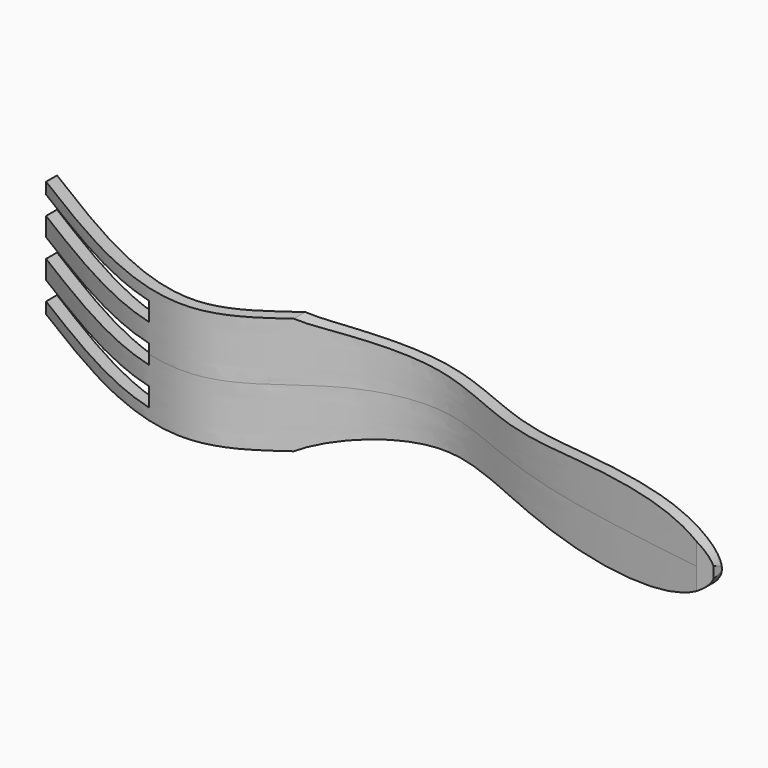
from build123d import *

# Parameters (mm, degrees)
F1_DEPTH = 12.7
F3_DEPTH = 25.4


# Not quite as in the source:
# - the dataset's text gives a spline's control points without its knots; the knots are read off the source's solid


with BuildPart() as f1:
    # F0 (on Top) → F1 (new body, symmetric)
    with BuildSketch(Plane.XY):
        with BuildLine():
            add(Edge.make_bspline(
                [(0, 0), (16.2681023426, -9.9387943725), (47.2246723498, -29.7831151482), (66.4369579208, -8.871840766), (90.9937113299, -1.8855664984), (116.1887648178, -16.7799469051), (146.2514664221, -20.7702417622), (163.4278756793, -23.4379916155)],
                knots=[0, 0, 0, 0, 0.2483058837, 0.4138785293, 0.5787286939, 0.7596256652, 1, 1, 1, 1], degree=3))
            Line((0, 0), (-1.3242090893, -2.1675032383))
            add(Edge.make_bspline(
                [(-1.3242090893, -2.1675032383), (2.7614631736, -4.6635937864), (9.136853643, -8.6121295805), (17.7262559137, -13.5899705503), (24.1194299019, -17.0078501308), (30.3765559587, -19.9378210176), (35.4147953662, -21.8277076646), (39.3127764924, -22.9151398196), (42.1656931351, -23.4919098932), (44.48213371, -23.7484534526), (46.2950869864, -23.8013359281), (47.6370394902, -23.7589266462), (48.9432550214, -23.6315977539), (50.6317203365, -23.3574905101), (52.6439135321, -22.8337162857), (54.9048810043, -21.9693426121), (57.7345292676, -20.5748674665), (60.9787182767, -18.5076431259), (63.9993416883, -16.3025670539), (66.3702951088, -14.6082956793), (68.14443987, -13.4065394694), (69.9302902852, -12.3121458679), (71.7789273461, -11.3143300486), (73.6737866655, -10.4200995816), (76.2525294434, -9.3737862154), (79.5499837318, -8.3545440034), (82.8865105773, -7.7567624188), (85.5439589903, -7.550857003), (87.5242249392, -7.5371713536), (89.4792915182, -7.667939484), (92.0667291299, -8.0436611912), (95.3527769387, -8.8658101088), (99.4476605789, -10.3024836387), (103.7644660516, -12.0561632537), (108.3706613255, -13.9763624934), (112.5069019539, -15.5824689852), (116.0392041879, -16.7871700333), (119.6906211821, -17.9104201543), (124.4593658972, -19.1816760405), (130.4643020599, -20.5322371053), (136.7041743745, -21.7458807941), (143.1310192089, -22.8586278685), (151.8841155603, -24.2548365718), (158.581573288, -25.2557425678), (163.0380499938, -25.9478991705)],
                knots=[0, 0, 0, 0, 0.0625, 0.09375, 0.125, 0.15625, 0.1875, 0.203125, 0.21875, 0.234375, 0.2421875, 0.25, 0.2578125, 0.265625, 0.28125, 0.296875, 0.3125, 0.34375, 0.375, 0.390625, 0.40625, 0.421875, 0.4375, 0.453125, 0.46875, 0.5, 0.53125, 0.546875, 0.5625, 0.578125, 0.59375, 0.625, 0.65625, 0.6875, 0.71875, 0.75, 0.765625, 0.78125, 0.8125, 0.84375, 0.875, 0.90625, 0.9375, 1, 1, 1, 1], degree=3))
            Line((163.0380499938, -25.9478991705), (163.4278756793, -23.4379916155))
        make_face()
    extrude(amount=F1_DEPTH, both=True)

    # F2 (on Front) → F3 (intersect)
    with BuildSketch(Plane.XZ):
        with BuildLine():
            Line((38.1, 2.0717850421), (38.1, 0))
            Line((38.1, 0), (38.1, -2.0717850421))
            Line((38.1, -2.0717850421), (0, -2.0717850421))
            Line((0, -2.0717850421), (0, -6.148728542))
            Line((0, -6.148728542), (38.1, -6.148728542))
            Line((38.1, -6.148728542), (38.1, -10.2256704122))
            Line((38.1, -10.2256704122), (0, -10.2256704122))
            Line((0, -10.2256704122), (0, -13.2833784446))
            Line((0, -13.2833784446), (63.5, -13.2833784446))
            add(Edge.make_bspline(
                [(63.5, -13.2833784446), (67.87038923, -9.7329119382), (103.5336972585, -4.9202314952), (125.3535669841, -8.8979314763), (154.1085600691, -9.4065150403), (163.4278756793, -2.4802493233), (163.4278756793, 0)],
                knots=[0, 0, 0, 0, 0.3081673451, 0.569189549, 0.8347896948, 1, 1, 1, 1], degree=3))
            add(Edge.make_bspline(
                [(63.5, 13.2833784446), (67.87038923, 9.7329119382), (103.5336972585, 4.9202314952), (125.3535669841, 8.8979314763), (154.1085600691, 9.4065150403), (163.4278756793, 2.4802493233), (163.4278756793, 0)],
                knots=[0, 0, 0, 0, 0.3081673451, 0.569189549, 0.8347896948, 1, 1, 1, 1], degree=3))
            Line((63.5, 13.2833784446), (0, 13.2833784446))
            Line((0, 13.2833784446), (0, 10.2256704122))
            Line((0, 10.2256704122), (38.1, 10.2256704122))
            Line((38.1, 10.2256704122), (38.1, 6.148728542))
            Line((38.1, 6.148728542), (0, 6.148728542))
            Line((0, 6.148728542), (0, 2.0717850421))
            Line((0, 2.0717850421), (38.1, 2.0717850421))
        make_face()
    extrude(amount=F3_DEPTH, mode=Mode.INTERSECT)


solid = f1.part
